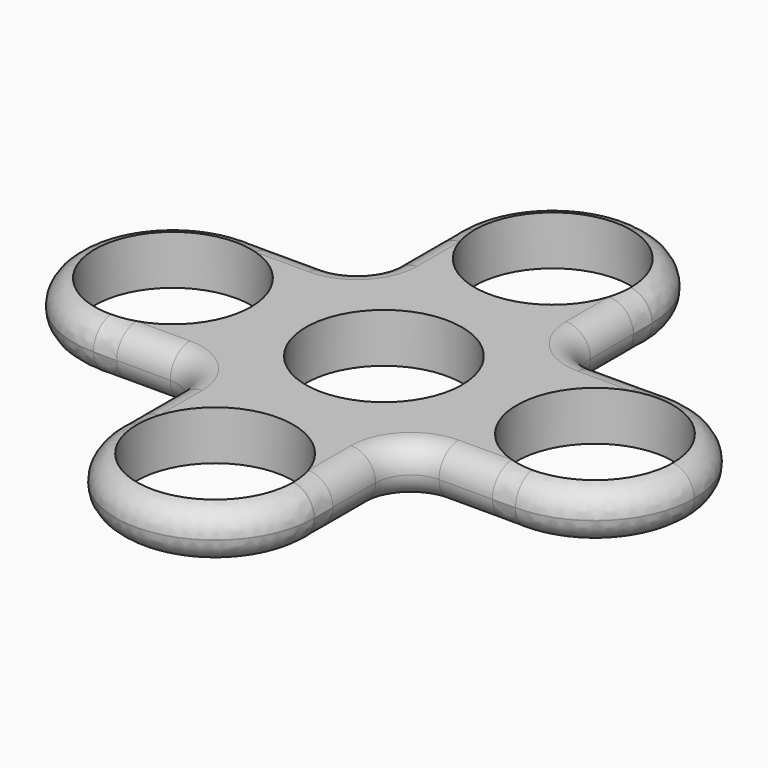
from build123d import *

# Parameters (mm, degrees)
F0_R     = 11.1
F1_DEPTH = 7
F2_R     = 5
F3_R     = 3.49999


# Not quite as in the source:
# - a fillet or chamfer is up to 0.001 mm smaller than in the source, because OpenCascade refuses the exact size


with BuildPart() as f1:
    # F0 (on Top) → F1 (new body)
    with BuildSketch(Plane.XY):
        with BuildLine():
            Line((14.1, 14.1), (14.1, 30))
            ThreePointArc((14.1, 30), (0, 44.1), (-14.1, 30))
            Line((-14.1, 30), (-14.1, 14.1))
            Line((-14.1, 14.1), (-30, 14.1))
            ThreePointArc((-30, 14.1), (-44.1, 0), (-30, -14.1))
            Line((-30, -14.1), (-14.1, -14.1))
            Line((-14.1, -14.1), (-14.1, -30))
            ThreePointArc((-14.1, -30), (0, -44.1), (14.1, -30))
            Line((14.1, -30), (14.1, -14.1))
            Line((14.1, -14.1), (30, -14.1))
            ThreePointArc((30, -14.1), (44.1, 0), (30, 14.1))
            Line((30, 14.1), (14.1, 14.1))
        make_face()
        with Locations((0, -30)):
            Circle(F0_R, mode=Mode.SUBTRACT)
        with Locations((-30, 0)):
            Circle(F0_R, mode=Mode.SUBTRACT)
        Circle(F0_R, mode=Mode.SUBTRACT)
        with Locations((30, 0)):
            Circle(F0_R, mode=Mode.SUBTRACT)
        with Locations((0, 30)):
            Circle(F0_R, mode=Mode.SUBTRACT)
    extrude(amount=F1_DEPTH)

    # F2
    f2_edges = [f1.edges().sort_by_distance(p)[0] for p in [
        (14.1, 14.1, 3.5),
        (-14.1, 14.1, 3.5),
        (-14.1, -14.1, 3.5),
        (14.1, -14.1, 3.5),
    ]]
    fillet(f2_edges, radius=F2_R)

    # F3 (radius 3.5 in the source; OpenCascade refuses exactly that, so slightly less here)
    f3_edges = [f1.edges().sort_by_distance(p)[0] for p in [
        (24.55, -14.1, 7),
        (44.1, 0, 0),
    ]]
    fillet(f3_edges, radius=F3_R)


solid = f1.part
